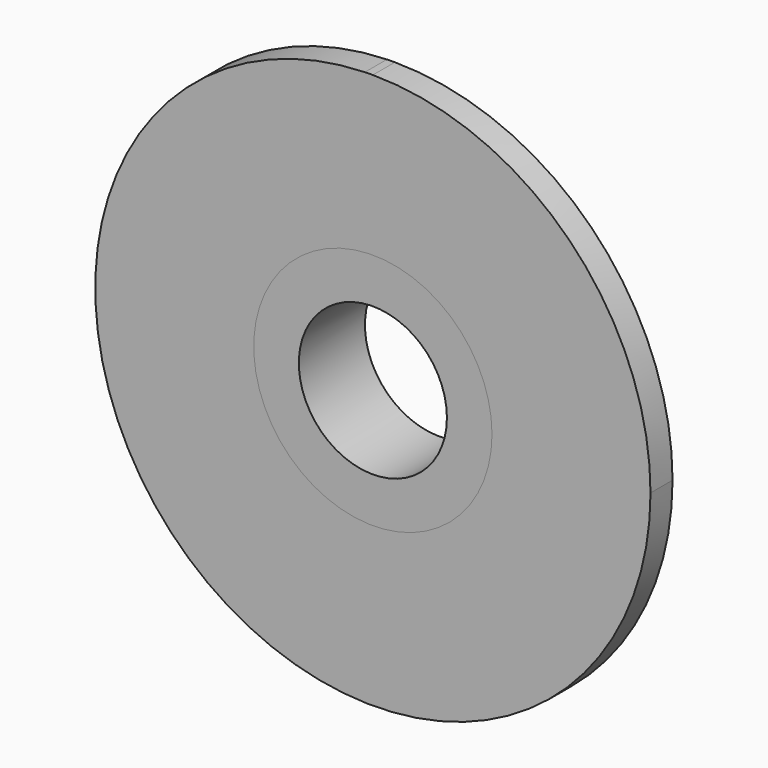
from build123d import *

# Parameters (mm, degrees)
F0_R     = 21.619902501
F0_R_2   = 13.4368376744
F1_DEPTH = 15
F2_DEPTH = 5


# Not quite as in the source:
# - the program builds the solid bodies; features that only make, move or delete a surface that nothing else refers to are left out


with BuildPart() as f1:
    # F0 (on Front) → F1 (new body)
    with BuildSketch(Plane.XZ):
        Circle(F0_R)
        Circle(F0_R_2, mode=Mode.SUBTRACT)
    extrude(amount=-F1_DEPTH)


with BuildPart() as f2:
    # F0 (on Front) → F2 (new body)
    with BuildSketch(Plane.XZ):
        with BuildLine():
            ThreePointArc((-1.4483617852, 50.3637455404), (-35.1114620527, -36.1357143176), (50.3845672475, 0))
            ThreePointArc((50.3845672475, 0), (35.6272691679, 35.6272691679), (0, 50.3845672475))
            Line((0, 50.3845672475), (-1.4483617852, 50.3637455404))
        make_face()
        Circle(F0_R, mode=Mode.SUBTRACT)
        with BuildLine():
            Line((-1.4483617852, 50.3637455404), (0, 50.3845672475))
            ThreePointArc((0, 50.3845672475), (-0.7242557221, 50.3793615518), (-1.4483617852, 50.3637455404))
        make_face()
    extrude(amount=-F2_DEPTH)


solid = Compound([f1.part, f2.part])
